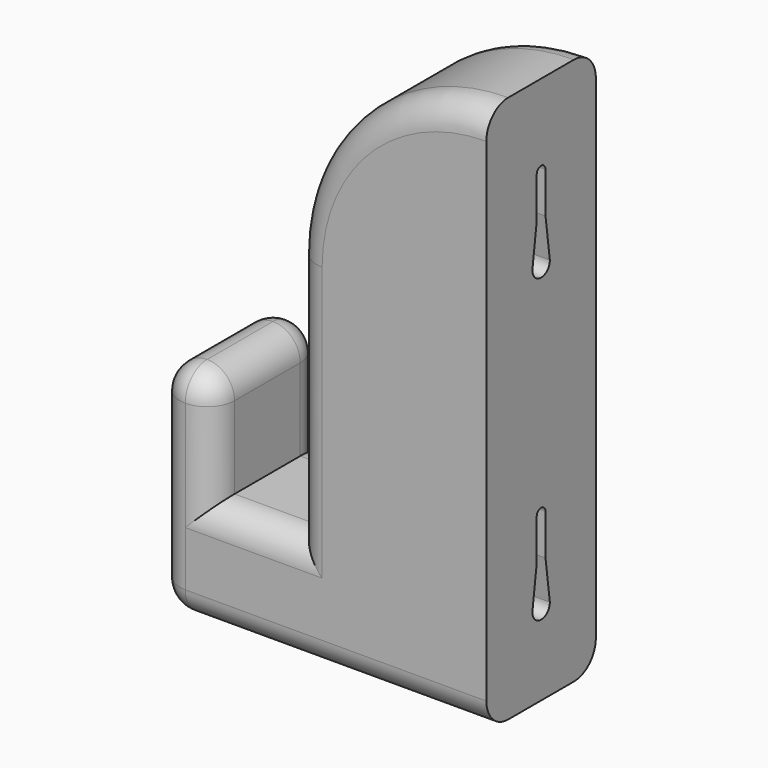
from build123d import *

# Parameters (mm, degrees)
F1_DEPTH    = 12.5
F2_R        = 4.99999
F3_T1_DEPTH = 25
F3_T4_ANGLE = 90
F3_T6_ANGLE = 90
F5_DEPTH    = 10
F7_DEPTH    = 5
F8_R        = 2


# Not quite as in the source:
# - a fillet or chamfer that OpenCascade refuses, or shapes differently, is made with other operations: its cross-section is extruded or revolved along the edge and cut away or added
# - a fillet or chamfer is up to 0.001 mm smaller than in the source, because OpenCascade refuses the exact size


with BuildPart() as f1:
    # F0 (on Front) → F1 (new body, symmetric)
    with BuildSketch(Plane.XZ):
        Polygon((-30, 40), (-30, 0), (30, 0), (30, 100), (-5, 100), (-5, 20), (-20, 20), (-20, 40), align=None)
    extrude(amount=F1_DEPTH, both=True)

    # F2 (radius 5 in the source; OpenCascade refuses exactly that, so slightly less here)
    f2_edges = [f1.edges().sort_by_distance(p)[0] for p in [
        (-30, 0, 40),
        (-30, 0, 0),
        (-20, 0, 40),
        (-12.5, -12.5, 20),
        (-12.5, 12.5, 20),
        (-30, -12.5, 20),
        (-20, -12.5, 30),
        (-25, -12.5, 40),
        (-25, 12.5, 40),
        (-30, 12.5, 20),
        (-20, 12.5, 30),
        (0, -12.5, 0),
        (0, 12.5, 0),
        (-5, -12.5, 60),
        (-5, 12.5, 60),
        (12.5, -12.5, 100),
        (12.5, 12.5, 100),
    ]]
    fillet(f2_edges, radius=F2_R)

    # F3: fillet of radius 35 on 1 edges, made by hand

    # F3_s2 → F3_t1 (cut)
    with BuildSketch(Plane.XZ.offset(-12.5)):
        with BuildLine():
            ThreePointArc((30, 100), (5.2512626585, 89.7487373415), (-5, 65))
            Line((-5, 65), (-5, 100))
            Line((-5, 100), (30, 100))
        make_face()
    extrude(amount=F3_T1_DEPTH, mode=Mode.SUBTRACT)

    # F3_s3 → F3_t4 (revolve, cut)
    with BuildSketch(Plane.XY.offset(65)):
        with BuildLine():
            ThreePointArc((-1e-05, 12.5), (-3.5355368349, 11.0355368349), (-5, 7.50001))
            Line((-5, 7.50001), (-5, 12.5))
            Line((-5, 12.5), (-1e-05, 12.5))
        make_face()
    revolve(axis=Axis((30, 12.5, 65), (0, 1, 0)), revolution_arc=F3_T4_ANGLE, mode=Mode.SUBTRACT)

    # F3_s5 → F3_t6 (revolve, cut)
    with BuildSketch(Plane.YZ.offset(30)):
        with BuildLine():
            ThreePointArc((-12.5, 95.00001), (-11.0355368349, 98.5355368349), (-7.50001, 100))
            Line((-7.50001, 100), (-12.5, 100))
            Line((-12.5, 100), (-12.5, 95.00001))
        make_face()
    revolve(axis=Axis((30, -12.5, 65), (0, -1, 0)), revolution_arc=F3_T6_ANGLE, mode=Mode.SUBTRACT)

    # F4 (on face) → F5 (cut)
    with BuildSketch(Plane.YZ.offset(30)):
        with BuildLine():
            ThreePointArc((-2, 15), (0, 13), (2, 15))
            Line((2, 15), (2, 30))
            ThreePointArc((2, 30), (0, 32), (-2, 30))
            Line((-2, 30), (-2, 15))
        make_face()
        with BuildLine():
            ThreePointArc((-2, 70), (0, 68), (2, 70))
            Line((2, 70), (2, 85))
            ThreePointArc((2, 85), (0, 87), (-2, 85))
            Line((-2, 85), (-2, 70))
        make_face()
    extrude(amount=-F5_DEPTH, mode=Mode.SUBTRACT)

    # F6 (on face) → F7 (join)
    with BuildSketch(Plane.YZ.offset(30)):
        with BuildLine():
            ThreePointArc((-1, 30), (0, 31), (1, 30))
            Line((1, 30), (1, 22.5))
            Line((1, 22.5), (2, 15))
            Line((2, 15), (2, 30))
            ThreePointArc((2, 30), (0, 32), (-2, 30))
            Line((-2, 30), (-2, 15))
            Line((-2, 15), (-1, 22.5))
            Line((-1, 22.5), (-1, 30))
        make_face()
        with BuildLine():
            Line((1, 85), (1, 77.5))
            Line((1, 77.5), (2, 70))
            Line((2, 70), (2, 85))
            ThreePointArc((2, 85), (0, 87), (-2, 85))
            Line((-2, 85), (-2, 70))
            Line((-2, 70), (-1, 77.5))
            Line((-1, 77.5), (-1, 85))
            ThreePointArc((-1, 85), (0, 86), (1, 85))
        make_face()
    extrude(amount=-F7_DEPTH)

    # F8
    f8_edges = [f1.edges().sort_by_distance(p)[0] for p in [
        (20, 0, 13),
        (20, 2, 22.5),
        (20, 0, 32),
        (20, -2, 22.5),
        (20, 0, 68),
        (20, 2, 77.5),
        (20, 0, 87),
        (20, -2, 77.5),
    ]]
    fillet(f8_edges, radius=F8_R)


solid = f1.part
